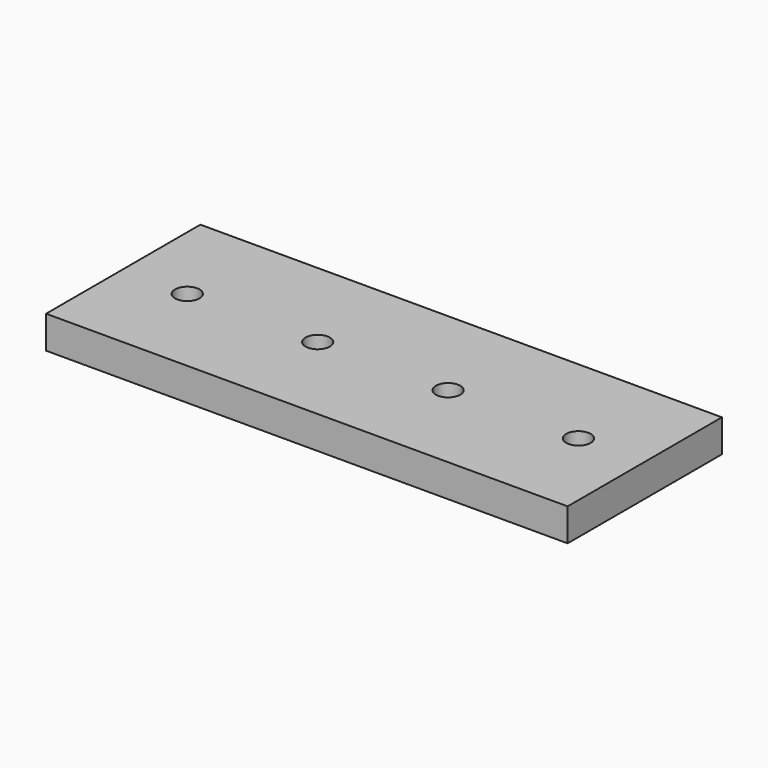
from build123d import *

# Parameters (mm, degrees)
F1_R     = 2.38125
F2_DEPTH = 6.35


# Not quite as in the source:
# - a length typed as a fraction of an inch, garbled in the dataset ("3 / 203.2 mm" for 3/8 in), is restored


with BuildPart() as f2:
    # F1 (on Top) → F2 (new body)
    with BuildSketch(Plane.XY):
        Polygon((101.6, 25.4093351929), (0, 25.4093351929), (0, 0), (0, -12.1591184288), (101.6, -12.1591184288), (101.6, 0.0093351929), align=None)
        with Locations((12.7, 6.35)):
            Circle(F1_R, mode=Mode.SUBTRACT)
        with Locations((38.1, 6.35)):
            Circle(F1_R, mode=Mode.SUBTRACT)
        with Locations((63.5, 6.35)):
            Circle(F1_R, mode=Mode.SUBTRACT)
        with Locations((88.9, 6.35)):
            Circle(F1_R, mode=Mode.SUBTRACT)
    extrude(amount=F2_DEPTH)


solid = f2.part
